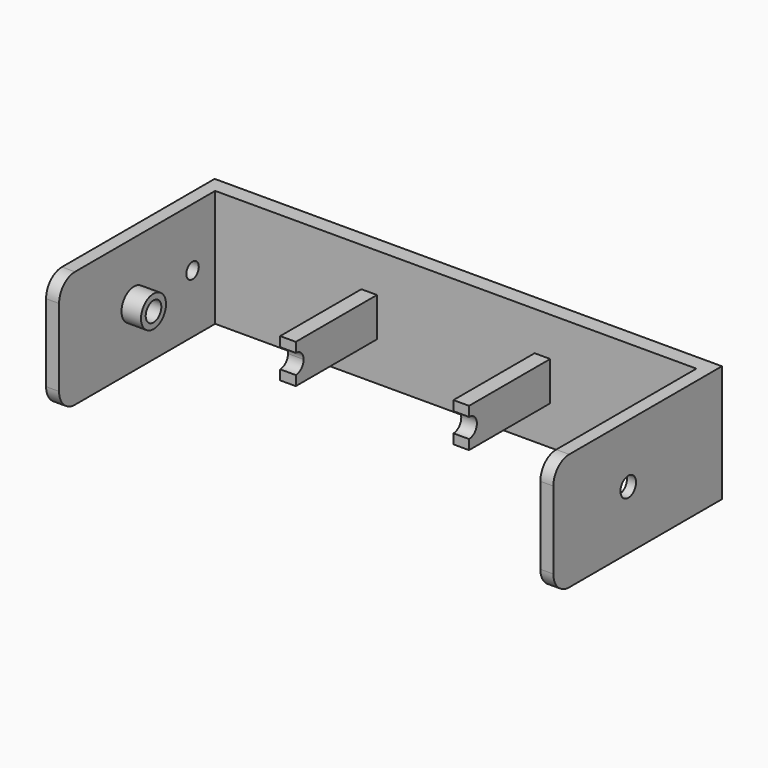
from build123d import *
from build123d import SkipClean  # not in build123d's __all__

# Parameters (mm, degrees)
F0_W      = 130
F0_H      = 30
F1_DEPTH  = 4
F2_W      = 3.3338604867
F2_H      = 30
F3_DEPTH  = 50
F4_R      = 5.08
F5_R      = 2.5
F6_DEPTH  = 137.16
F7_R      = 4
F7_R_2    = 2.5
F8_DEPTH  = 5
F9_W      = 15
F9_H      = 15
F9_R      = 2.5
F10_DEPTH = 1
F11_W     = 4
F11_H     = 10
F12_DEPTH = 26.0096
F14_DEPTH = 14.224
F16_DEPTH = 6.096
F17_R     = 1.9939
F18_DEPTH = 25.4


# Not quite as in the source:
# - after a boolean that leaves OpenCascade's solid faulty, fix() repairs it
# - a feature names something its author has since deleted; it is built from what else it names


with BuildPart() as f1:
    # F0 (on Front) → F1 (new body)
    with BuildSketch(Plane.XZ):
        Rectangle(F0_W, F0_H)
    extrude(amount=F1_DEPTH)

    # F2 (on face) → F3 (join)
    with BuildSketch(Plane.XZ.offset(4)):
        with Locations((-63.3330697566, 0)):
            Rectangle(F2_W, F2_H)
        with Locations((63.3330697566, 0)):
            Rectangle(F2_W, F2_H)
    extrude(amount=F3_DEPTH)

    # F4
    f4_edges = [f1.edges().sort_by_distance(p)[0] for p in [
        (63.33307, -54, 15),
        (63.33307, -54, -15),
        (-63.33307, -54, -15),
        (-63.33307, -54, 15),
    ]]
    fillet(f4_edges, radius=F4_R)

    # F5 (on face) → F6 (cut)
    with BuildSketch(Plane(origin=(-65, 0, 0), x_dir=(0, -1, 0), z_dir=(-1, 0, 0))):
        with Locations((30, 0)):
            Circle(F5_R)
    extrude(amount=-F6_DEPTH, mode=Mode.SUBTRACT)

    # F7 (on face) → F8 (join)
    with BuildSketch(Plane.YZ.offset(-61.6661395133)):
        with Locations((-30, 0)):
            Circle(F7_R)
        with Locations((-30, 0)):
            Circle(F7_R_2, mode=Mode.SUBTRACT)
    with SkipClean():  # cleaning this boolean's faces spoils the solid; the shape is the same uncleaned
        extrude(amount=F8_DEPTH)

    # F9 (on face) → F10 (cut)
    with BuildSketch(Plane(origin=(61.6661395133, 0, 0), x_dir=(0, -1, 0), z_dir=(-1, 0, 0))):
        with Locations((30, 0)):
            Rectangle(F9_W, F9_H)
        with Locations((30, 0)):
            Circle(F9_R, mode=Mode.SUBTRACT)
    extrude(amount=-F10_DEPTH, mode=Mode.SUBTRACT)

    add(f1.part.fix(), mode=Mode.REPLACE)

    # F11 (on face) → F12 (join)
    with BuildSketch(Plane.XZ.offset(4)):
        with Locations((-22.1996698529, 0)):
            Rectangle(F11_W, F11_H)
        with Locations((22.1996698529, 0)):
            Rectangle(F11_W, F11_H)
    extrude(amount=F12_DEPTH)

    # F13 (on face) → F14 (cut)
    with BuildSketch(Plane.YZ.offset(-20.1996698529)):
        with BuildLine():
            ThreePointArc((-30.0096, -2.4999815679), (-28.2356304242, -1.7711578134), (-27.5, 0))
            ThreePointArc((-27.5, 0), (-28.2356304242, 1.7711578134), (-30.0096, 2.4999815679))
            Line((-30.0096, 2.4999815679), (-30.0096, -2.4999815679))
        make_face()
    extrude(amount=-F14_DEPTH, mode=Mode.SUBTRACT)

    # F15 (on face) → F16 (cut)
    with BuildSketch(Plane.YZ.offset(24.1996698529)):
        with BuildLine():
            Line((-30.0096, 2.4999815679), (-30.0096, -2.4999815679))
            ThreePointArc((-30.0096, -2.4999815679), (-27.5, 0), (-30.0096, 2.4999815679))
        make_face()
    extrude(amount=-F16_DEPTH, mode=Mode.SUBTRACT)

    # F17 (on face) → F18 (cut)
    with BuildSketch(Plane(origin=(-65, 0, 0), x_dir=(0, -1, 0), z_dir=(-1, 0, 0))):
        with Locations((11.25, 0)):
            Circle(F17_R)
    extrude(amount=-F18_DEPTH, mode=Mode.SUBTRACT)


solid = f1.part
